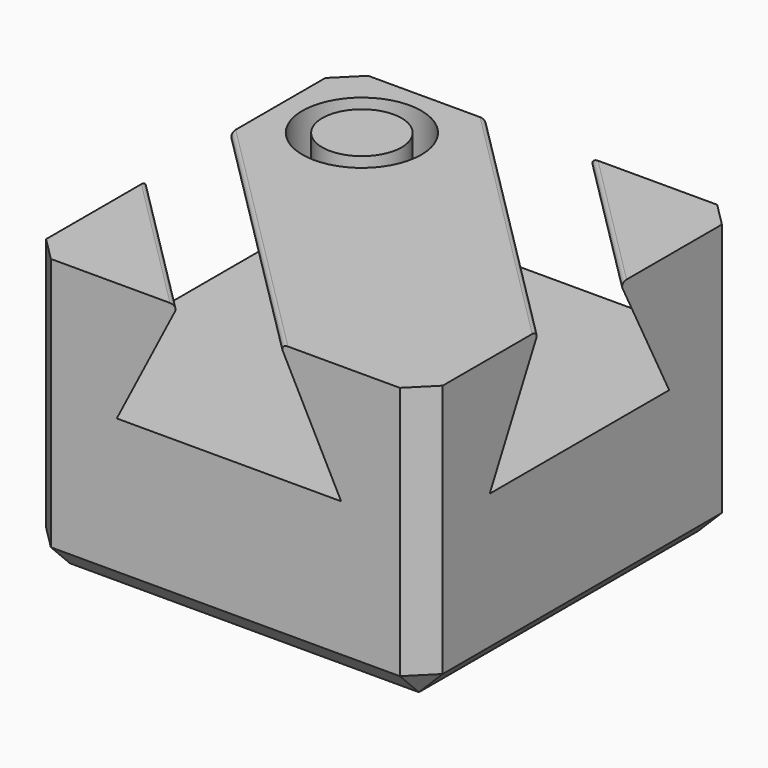
from build123d import *

# Parameters (mm, degrees)
F0_W     = 50
F0_H     = 50
F1_DEPTH = 35
F4_DEPTH = 74.8112648726
F6_SIZE  = 3
F7_R     = 0.5
F8_R     = 7.5
F8_R_2   = 5
F9_DEPTH = 13


# Not quite as in the source:
# - a pattern or mirror of a feature is missing from the dataset's text; its kind, count and spacing are read off the source's solid


with BuildPart() as f1:
    # F0 (on Top) → F1 (new body)
    with BuildSketch(Plane.XY):
        Rectangle(F0_W, F0_H)
    extrude(amount=F1_DEPTH)

    # F3 (on face) → F4 (cut)
    with BuildSketch(Plane(origin=(25, -25, 0), x_dir=(-0.7071067812, -0.7071067812, 0), z_dir=(-0.7071067812, 0.7071067812, 0))):
        Polygon((27.3553390593, 20), (21.8957855453, 35), (12.8148925733, 35), (7.3553390593, 20), align=None)
    f4 = extrude(amount=F4_DEPTH, mode=Mode.SUBTRACT)

    # F4_copies: F4 across plane
    add(f4.mirror(Plane(origin=(0, 0, 0), x_dir=(0.7071067812, -0.7071067812, 0), z_dir=(0.7071067812, 0.7071067812, 0))), mode=Mode.SUBTRACT)

    # F6
    f6_edges = [f1.edges().sort_by_distance(p)[0] for p in [
        (25, 0, 0),
        (0, -25, 0),
        (-25, 0, 0),
        (0, 25, 0),
        (25, -25, 17.5),
        (-25, -25, 17.5),
        (-25, 25, 17.5),
        (25, 25, 17.5),
    ]]
    chamfer(f6_edges, length=F6_SIZE)

    # F7
    f7_edges = [f1.edges().sort_by_distance(p)[0] for p in [
        (-15.482658, -15.482658, 35),
        (-9.061497, -9.061497, 35),
        (9.061497, 9.061497, 35),
        (15.482658, 15.482658, 35),
    ]]
    fillet(f7_edges, radius=F7_R)

    # F8 (on face) → F9 (cut)
    with BuildSketch(Plane.XY.offset(35)):
        with Locations((-14.8947280353, 15.1347092162)):
            Circle(F8_R)
        with Locations((-14.8947280353, 15.1347092162)):
            Circle(F8_R_2, mode=Mode.SUBTRACT)
    extrude(amount=-F9_DEPTH, mode=Mode.SUBTRACT)


solid = f1.part
